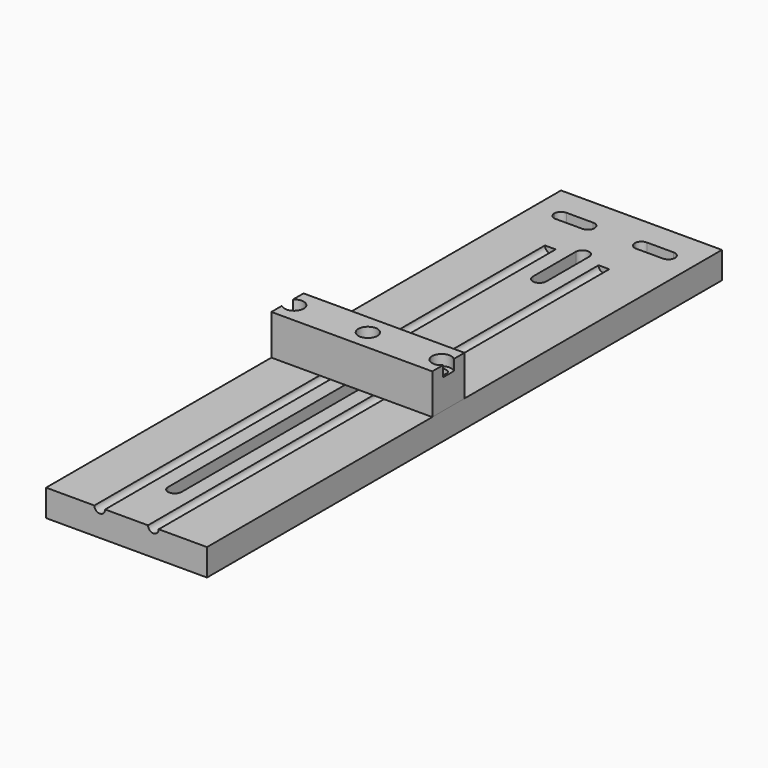
from build123d import *

# Parameters (mm, degrees)
F0_W            = 120
F0_H            = 20
F1_DEPTH        = 480
F3_DEPTH        = 20.001
F5_DEPTH        = 6.1
F7_DEPTH        = 20.001
F9_DEPTH        = 9
F11_DEPTH       = 420
F12_W           = 120
F12_H           = 30
F13_DEPTH       = 30
F15_D           = 7.4
F15_DEPTH       = 50
F15_CBORE_D     = 14.25
F15_CBORE_DEPTH = 8
F15_TIP         = 2.2231842904


# Not quite as in the source:
# - a feature names something its author has since deleted; it is built from what else it names


with BuildPart() as f1:
    # F0 (on Front) → F1 (new body)
    with BuildSketch(Plane.XZ):
        with Locations((0, 10)):
            Rectangle(F0_W, F0_H)
    extrude(amount=-F1_DEPTH)

    # F2 (on face) → F3 (cut, through all)
    with BuildSketch(Plane.XY.offset(20)):
        with BuildLine():
            ThreePointArc((5, 245), (0, 250), (-5, 245))
            Line((-5, 245), (-5, 45))
            ThreePointArc((-5, 45), (0, 40), (5, 45))
            Line((5, 45), (5, 245))
        make_face()
        with BuildLine():
            ThreePointArc((5, 425), (0, 430), (-5, 425))
            Line((-5, 425), (-5, 385))
            ThreePointArc((-5, 385), (0, 380), (5, 385))
            Line((5, 385), (5, 425))
        make_face()
    extrude(amount=-F3_DEPTH, mode=Mode.SUBTRACT)

    # F4 (on face) → F5 (cut)
    with BuildSketch(Plane(origin=(0, 0, 0), x_dir=(1, 0, 0), z_dir=(0, 0, -1))):
        with BuildLine():
            Line((8, -245), (8, -45))
            ThreePointArc((8, -45), (0, -37), (-8, -45))
            Line((-8, -45), (-8, -245))
            ThreePointArc((-8, -245), (0, -253), (8, -245))
        make_face()
        with BuildLine():
            ThreePointArc((8, -385), (0, -377), (-8, -385))
            Line((-8, -385), (-8, -425))
            ThreePointArc((-8, -425), (0, -433), (8, -425))
            Line((8, -425), (8, -385))
        make_face()
    extrude(amount=-F5_DEPTH, mode=Mode.SUBTRACT)

    # F6 (on face) → F7 (cut, through all)
    with BuildSketch(Plane.XY.offset(20)):
        with BuildLine():
            ThreePointArc((-45, 455), (-43.5355339059, 451.4644660941), (-40, 450))
            Line((-40, 450), (-20, 450))
            ThreePointArc((-20, 450), (-16.4644660941, 451.4644660941), (-15, 455))
            ThreePointArc((-15, 455), (-16.4644660941, 458.5355339059), (-20, 460))
            Line((-20, 460), (-40, 460))
            ThreePointArc((-40, 460), (-43.5355339059, 458.5355339059), (-45, 455))
        make_face()
        with BuildLine():
            ThreePointArc((45, 455), (43.5355339059, 458.5355339059), (40, 460))
            Line((40, 460), (20, 460))
            ThreePointArc((20, 460), (16.4644660941, 458.5355339059), (15, 455))
            ThreePointArc((15, 455), (16.4644660941, 451.4644660941), (20, 450))
            Line((20, 450), (40, 450))
            ThreePointArc((40, 450), (43.5355339059, 451.4644660941), (45, 455))
        make_face()
    extrude(amount=-F7_DEPTH, mode=Mode.SUBTRACT)

    # F8 (on face) → F9 (cut)
    with BuildSketch(Plane(origin=(0, 0, 0), x_dir=(1, 0, 0), z_dir=(0, 0, -1))):
        with BuildLine():
            Line((-15, -447), (-50, -447))
            Line((-50, -447), (-50, -463))
            Line((-50, -463), (-15, -463))
            ThreePointArc((-15, -463), (-7, -455), (-15, -447))
        make_face()
        with BuildLine():
            Line((50, -447), (15, -447))
            ThreePointArc((15, -447), (7, -455), (15, -463))
            Line((15, -463), (50, -463))
            Line((50, -463), (50, -447))
        make_face()
    extrude(amount=-F9_DEPTH, mode=Mode.SUBTRACT)

    # F10 (on face) → F11 (cut)
    with BuildSketch(Plane.XZ):
        with BuildLine():
            ThreePointArc((-24, 20), (-20, 16), (-16, 20))
            Line((-16, 20), (-24, 20))
        make_face()
        with BuildLine():
            Line((24, 20), (16, 20))
            ThreePointArc((16, 20), (20, 16), (24, 20))
        make_face()
    extrude(amount=-F11_DEPTH, mode=Mode.SUBTRACT)


with BuildPart() as f13:
    # F12 (on face) → F13 (new body)
    with BuildSketch(Plane.XY.offset(20)):
        with Locations((0, 225)):
            Rectangle(F12_W, F12_H)
    extrude(amount=F13_DEPTH)

    # F15
    with Locations(Plane.XY.offset(50)):
        with Locations((-55, 225), (55, 225), (0, 225)):
            CounterBoreHole(F15_D / 2, F15_CBORE_D / 2, F15_CBORE_DEPTH, depth=F15_DEPTH)
            with Locations((0, 0, -(F15_DEPTH + F15_TIP / 2))):  # 118° drill point
                Cone(0, F15_D / 2, F15_TIP, mode=Mode.SUBTRACT)


solid = Compound([f1.part, f13.part])
